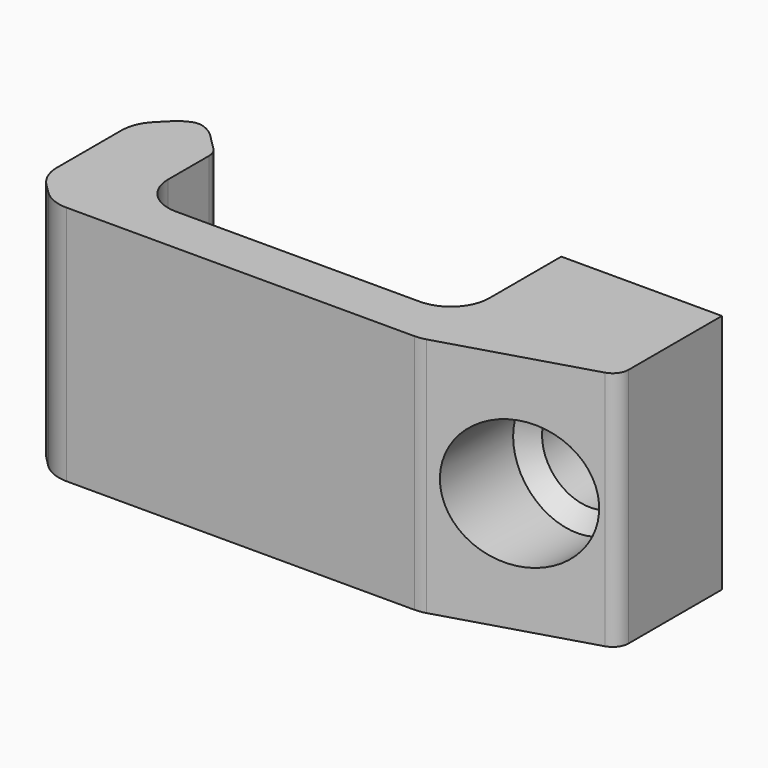
from build123d import *

# Parameters (mm, degrees)
F0_W        = 10
F0_H        = 8
F1_DEPTH    = 15
F2_R        = 4
F2_R_2      = 3
F3_DEPTH    = 25
F4_DEPTH    = 5
F5_SIZE     = 0.99999
F6_SIZE     = 2
F7_T1_DEPTH = 15
F7_T3_DEPTH = 19.9705627485
F7_T5_DEPTH = 16.7612260356
F8_R        = 1


# Not quite as in the source:
# - a fillet or chamfer that OpenCascade refuses, or shapes differently, is made with other operations: its cross-section is extruded or revolved along the edge and cut away or added
# - a fillet or chamfer is up to 0.001 mm smaller than in the source, because OpenCascade refuses the exact size


with BuildPart() as f1:
    # F0 (on Top) → F1 (new body)
    with BuildSketch(Plane.XY):
        Polygon((20, -8), (0, -8), (0, 0), (-5, 0), (-5, -11), (20, -11), align=None)
        with Locations((25, -4)):
            Rectangle(F0_W, F0_H)
        Polygon((30, -8), (20, -8), (20, -11), align=None)
    extrude(amount=F1_DEPTH)

    # F2 (on face) → F3 (cut)
    with BuildSketch(Plane(origin=(0, 0, 0), x_dir=(-1, 0, 0), z_dir=(0, 1, 0))):
        with Locations((-25, 7.5)):
            Circle(F2_R)
        with Locations((-25, 7.5)):
            Circle(F2_R_2, mode=Mode.SUBTRACT)
        with Locations((-25, 7.5)):
            Circle(F2_R_2)
    extrude(amount=-F3_DEPTH, mode=Mode.SUBTRACT)

    # F2 (on face) → F4 (join)
    with BuildSketch(Plane(origin=(0, 0, 0), x_dir=(-1, 0, 0), z_dir=(0, 1, 0))):
        with Locations((-25, 7.5)):
            Circle(F2_R)
        with Locations((-25, 7.5)):
            Circle(F2_R_2, mode=Mode.SUBTRACT)
    extrude(amount=-F4_DEPTH)

    # F5 (size 1 in the source; OpenCascade refuses exactly that, so slightly less here)
    f5_edges = [f1.edges().sort_by_distance(p)[0] for p in [
        (28, -5, 7.5),
    ]]
    chamfer(f5_edges, length=F5_SIZE)

    # F6
    f6_edges = [f1.edges().sort_by_distance(p)[0] for p in [
        (-5, 0, 7.5),
        (0, 0, 7.5),
        (-5, -11, 7.5),
    ]]
    chamfer(f6_edges, length=F6_SIZE)

    # F7: fillet of radius 2.4 on 8 edges, made by hand

    # F7_s2 → F7_t1 (join)
    with BuildSketch(Plane.XY):
        with BuildLine():
            ThreePointArc((0, -5.6), (0.7029437252, -7.2970562748), (2.4, -8))
            Line((2.4, -8), (0, -8))
            Line((0, -8), (0, -5.6))
        make_face()
        with BuildLine():
            ThreePointArc((17.6, -8), (19.2970562748, -7.2970562748), (20, -5.6))
            Line((20, -5.6), (20, -8))
            Line((20, -8), (17.6, -8))
        make_face()
    extrude(amount=F7_T1_DEPTH)

    # F7_s4 → F7_t3 (cut)
    with BuildSketch(Plane.XY.offset(-2.4852813742)):
        with BuildLine():
            ThreePointArc((-1.2970562748, -0.7029437252), (-2.075672312, -0.182689122), (-2.9941125497, 0))
            Line((-2.9941125497, 0), (-2, 0))
            Line((-2, 0), (-1.2970562748, -0.7029437252))
        make_face()
        with BuildLine():
            ThreePointArc((-2.0058874503, 0), (-2.924327688, -0.182689122), (-3.7029437252, -0.7029437252))
            Line((-3.7029437252, -0.7029437252), (-3, 0))
            Line((-3, 0), (-2.0058874503, 0))
        make_face()
        with BuildLine():
            ThreePointArc((-4.2970562748, -1.2970562748), (-4.817310878, -2.075672312), (-5, -2.9941125497))
            Line((-5, -2.9941125497), (-5, -2))
            Line((-5, -2), (-4.2970562748, -1.2970562748))
        make_face()
        with BuildLine():
            ThreePointArc((-5, -8.0058874503), (-4.817310878, -8.924327688), (-4.2970562748, -9.7029437252))
            Line((-4.2970562748, -9.7029437252), (-5, -9))
            Line((-5, -9), (-5, -8.0058874503))
        make_face()
        with BuildLine():
            ThreePointArc((-3.7029437252, -10.2970562748), (-2.924327688, -10.817310878), (-2.0058874503, -11))
            Line((-2.0058874503, -11), (-3, -11))
            Line((-3, -11), (-3.7029437252, -10.2970562748))
        make_face()
    extrude(amount=F7_T3_DEPTH, mode=Mode.SUBTRACT)

    # F7_s6 → F7_t5 (cut)
    with BuildSketch(Plane.XY.offset(-0.8806130178)):
        with BuildLine():
            ThreePointArc((20.3373897182, -10.8987830845), (19.9962663401, -10.9745609492), (19.6477547929, -11))
            Line((19.6477547929, -11), (20, -11))
            Line((20, -11), (20.3373897182, -10.8987830845))
        make_face()
    extrude(amount=F7_T5_DEPTH, mode=Mode.SUBTRACT)

    # F8
    f8_edges = [f1.edges().sort_by_distance(p)[0] for p in [
        (-2.5, -0.051415, 7.5),
        (0, -2, 7.5),
        (30, -8, 7.5),
    ]]
    fillet(f8_edges, radius=F8_R)


solid = f1.part
